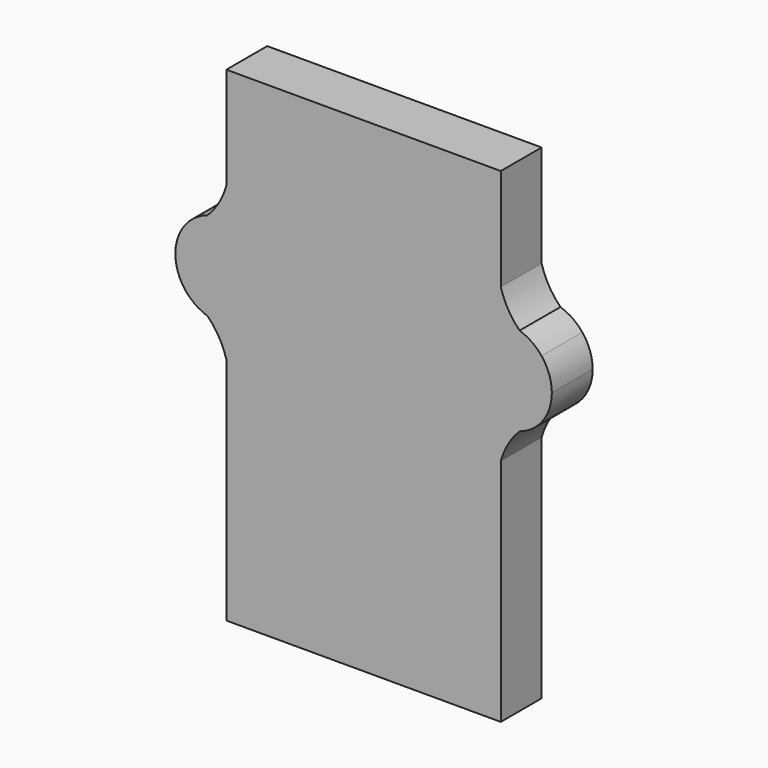
from build123d import *

# Parameters (mm, degrees)
F0_W     = 136.525
F0_H     = 241.3
F1_DEPTH = 25.4
F3_DEPTH = 25.4


with BuildPart() as f1:
    # F0 (on Front) → F1 (new body)
    with BuildSketch(Plane.XZ):
        Rectangle(F0_W, F0_H)
    extrude(amount=F1_DEPTH)

    # F2 (on face) → F3 (join)
    with BuildSketch(Plane.XZ.offset(25.4)):
        with BuildLine():
            ThreePointArc((77.6254340957, 53.8129340957), (71.9080698474, 61.2266782869), (68.2625, 69.85))
            Line((68.2625, 69.85), (68.2625, -6.35))
            ThreePointArc((68.2625, -6.35), (71.9080698474, 2.2733217131), (77.6254340957, 9.6870659043))
            ThreePointArc((77.6254340957, 9.6870659043), (82.7346936877, 13.9409024845), (88.5302033496, 17.1984670639))
            ThreePointArc((88.5302033496, 17.1984670639), (92.3418278085, 24.0349565831), (93.6625, 31.75))
            ThreePointArc((93.6625, 31.75), (92.3418278085, 39.4650434169), (88.5302033496, 46.3015329361))
            ThreePointArc((88.5302033496, 46.3015329361), (82.7346936877, 49.5590975155), (77.6254340957, 53.8129340957))
        make_face()
        with BuildLine():
            ThreePointArc((88.5302033496, 46.3015329361), (83.6252121519, 50.8519186766), (77.6254340957, 53.8129340957))
            ThreePointArc((77.6254340957, 53.8129340957), (82.7346936877, 49.5590975155), (88.5302033496, 46.3015329361))
        make_face()
        with BuildLine():
            ThreePointArc((88.5302033496, 17.1984670639), (82.7346936877, 13.9409024845), (77.6254340957, 9.6870659043))
            ThreePointArc((77.6254340957, 9.6870659043), (83.6252121519, 12.6480813234), (88.5302033496, 17.1984670639))
        make_face()
    extrude(amount=-F3_DEPTH)

    # F4: F1 across plane


with BuildPart() as f1_1:
    add(f1.part)
    add(f1.part.mirror(Plane.YZ))


solid = f1_1.part
